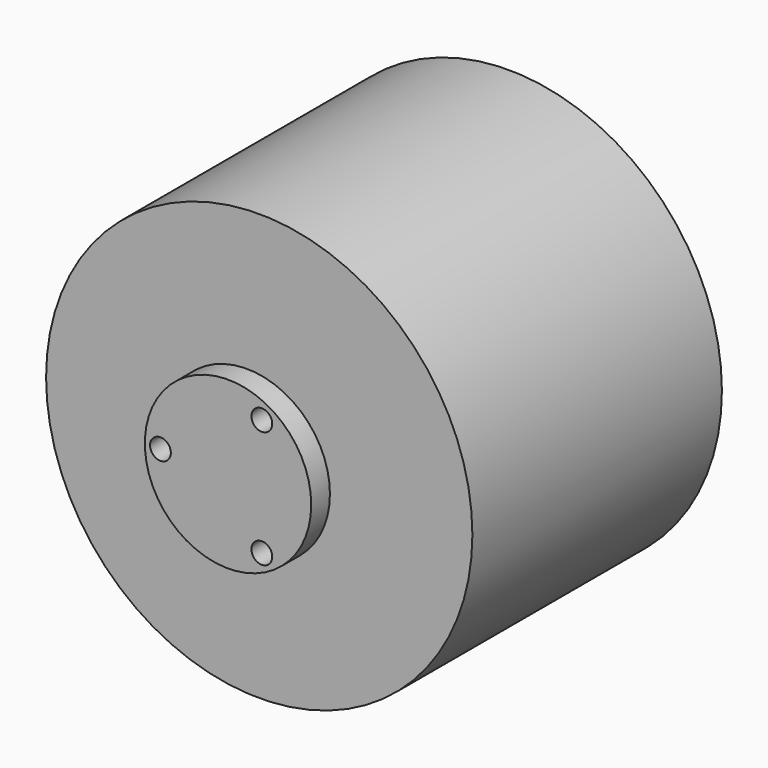
from build123d import *

# Parameters (mm, degrees)
F0_R            = 41
F1_DEPTH        = 30
F1_DEPTH_BACK   = 30
F2_R            = 10
F3_DEPTH        = 3
F4_R            = 16
F5_DEPTH        = 4.5
F7_D            = 4
F7_DEPTH        = 5
F7_TIP          = 1.2017212381
F7_COPIES_COUNT = 3


# Not quite as in the source:
# - a pattern or mirror of a feature is missing from the dataset's text; its kind, count and spacing are read off the source's solid


with BuildPart() as f1:
    # F0 (on Front) → F1 (new body, two sides)
    with BuildSketch(Plane.XZ) as f1_sk:
        Circle(F0_R)
    extrude(amount=F1_DEPTH)
    extrude(f1_sk.sketch, amount=-F1_DEPTH_BACK)

    # F2 (on face) → F3 (join)
    with BuildSketch(Plane.XZ.offset(30)):
        Circle(F2_R)
    extrude(amount=F3_DEPTH)

    # F4 (on face) → F5 (join)
    with BuildSketch(Plane.XZ.offset(33)):
        Circle(F4_R)
    extrude(amount=F5_DEPTH)

    # F7
    with Locations(Plane.XZ.offset(37.5)):
        with Locations((-13, 0)):
            f7 = Hole(F7_D / 2, depth=F7_DEPTH)
            with Locations((0, 0, -(F7_DEPTH + F7_TIP / 2))):  # 118° drill point
                Cone(0, F7_D / 2, F7_TIP, mode=Mode.SUBTRACT)

    # F7_copies: F7 ×3 about axis
    f7_copies_axis = Axis((0, 0, 0), (0, 1, 0))
    for i in range(1, F7_COPIES_COUNT):
        add(f7.rotate(f7_copies_axis, i * 360 / F7_COPIES_COUNT), mode=Mode.SUBTRACT)


solid = f1.part
